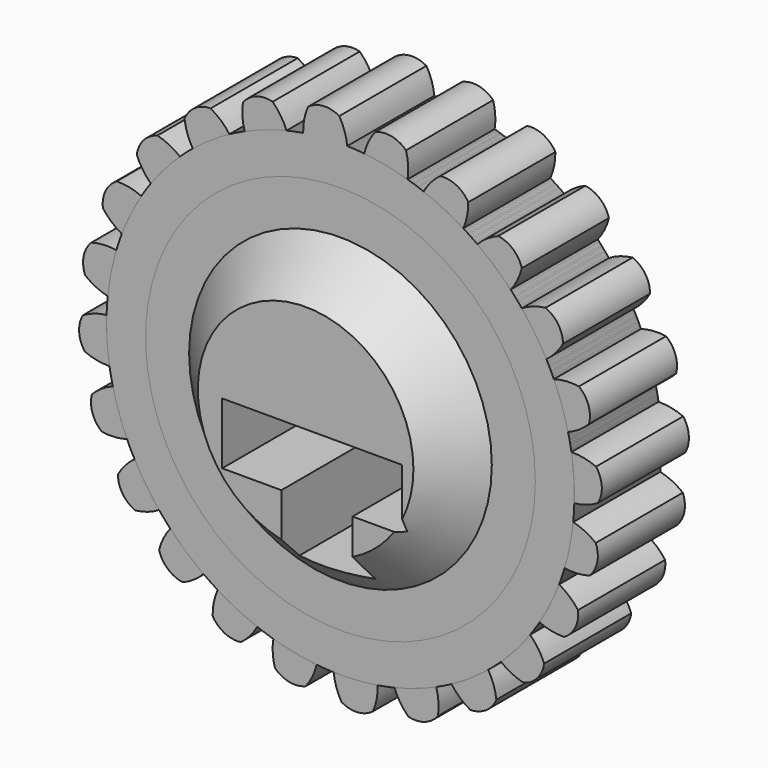
from build123d import *

# Parameters (mm, degrees)
F0_R     = 34.7544830967
F1_DEPTH = 25
F2_COUNT = 24
F3_DEPTH = 25
F4_DEPTH = 35


# Not quite as in the source:
# - a fillet or chamfer that OpenCascade refuses, or shapes differently, is made with other operations: its cross-section is extruded or revolved along the edge and cut away or added


with BuildPart() as f1:
    # F0 (on Front) → F1 (new body)
    with BuildSketch(Plane.XZ):
        with BuildLine():
            ThreePointArc((-8.5592843012, 53.0347479795), (-3.5135215054, 53.6059792153), (1.5636347284, 53.6982391465))
            ThreePointArc((1.5636347284, 53.6982391465), (0.9452694669, 56.5284341195), (-0.2671070692, 59.1595027839))
            ThreePointArc((-0.2671070692, 59.1595027839), (-3.9330463258, 60.0066910843), (-7.4570427008, 58.6882495052))
            ThreePointArc((-7.4570427008, 58.6882495052), (-8.3156238134, 55.9214431052), (-8.5592843012, 53.0347479795))
        make_face()
        with BuildLine():
            ThreePointArc((-8.5592843012, 53.0347479795), (-34.8291008286, -40.9008505593), (53.721, 0))
            ThreePointArc((53.721, 0), (38.5353465162, 37.4295726649), (1.5636347284, 53.6982391465))
            ThreePointArc((1.5636347284, 53.6982391465), (-3.5135215054, 53.6059792153), (-8.5592843012, 53.0347479795))
        make_face()
        Circle(F0_R, mode=Mode.SUBTRACT)
    extrude(amount=F1_DEPTH)


with BuildPart() as f2_1:
    # F2: instance of F1
    add(f1.part.rotate(Axis((0, 0, 0), (0, 1, 0)), 1 * 360 / F2_COUNT))


with BuildPart() as f2_2:
    # F2: instance of F1
    add(f1.part.rotate(Axis((0, 0, 0), (0, 1, 0)), 2 * 360 / F2_COUNT))


with BuildPart() as f2_3:
    # F2: instance of F1
    add(f1.part.rotate(Axis((0, 0, 0), (0, 1, 0)), 3 * 360 / F2_COUNT))


with BuildPart() as f2_4:
    # F2: instance of F1
    add(f1.part.rotate(Axis((0, 0, 0), (0, 1, 0)), 4 * 360 / F2_COUNT))


with BuildPart() as f2_5:
    # F2: instance of F1
    add(f1.part.rotate(Axis((0, 0, 0), (0, 1, 0)), 5 * 360 / F2_COUNT))


with BuildPart() as f2_6:
    # F2: instance of F1
    add(f1.part.rotate(Axis((0, 0, 0), (0, 1, 0)), 6 * 360 / F2_COUNT))


with BuildPart() as f2_7:
    # F2: instance of F1
    add(f1.part.rotate(Axis((0, 0, 0), (0, 1, 0)), 7 * 360 / F2_COUNT))


with BuildPart() as f2_8:
    # F2: instance of F1
    add(f1.part.rotate(Axis((0, 0, 0), (0, 1, 0)), 8 * 360 / F2_COUNT))


with BuildPart() as f2_9:
    # F2: instance of F1
    add(f1.part.rotate(Axis((0, 0, 0), (0, 1, 0)), 9 * 360 / F2_COUNT))


with BuildPart() as f2_10:
    # F2: instance of F1
    add(f1.part.rotate(Axis((0, 0, 0), (0, 1, 0)), 10 * 360 / F2_COUNT))


with BuildPart() as f2_11:
    # F2: instance of F1
    add(f1.part.rotate(Axis((0, 0, 0), (0, 1, 0)), 11 * 360 / F2_COUNT))


with BuildPart() as f2_12:
    # F2: instance of F1
    add(f1.part.rotate(Axis((0, 0, 0), (0, 1, 0)), 12 * 360 / F2_COUNT))


with BuildPart() as f2_13:
    # F2: instance of F1
    add(f1.part.rotate(Axis((0, 0, 0), (0, 1, 0)), 13 * 360 / F2_COUNT))


with BuildPart() as f2_14:
    # F2: instance of F1
    add(f1.part.rotate(Axis((0, 0, 0), (0, 1, 0)), 14 * 360 / F2_COUNT))


with BuildPart() as f2_15:
    # F2: instance of F1
    add(f1.part.rotate(Axis((0, 0, 0), (0, 1, 0)), 15 * 360 / F2_COUNT))


with BuildPart() as f2_16:
    # F2: instance of F1
    add(f1.part.rotate(Axis((0, 0, 0), (0, 1, 0)), 16 * 360 / F2_COUNT))


with BuildPart() as f2_17:
    # F2: instance of F1
    add(f1.part.rotate(Axis((0, 0, 0), (0, 1, 0)), 17 * 360 / F2_COUNT))


with BuildPart() as f2_18:
    # F2: instance of F1
    add(f1.part.rotate(Axis((0, 0, 0), (0, 1, 0)), 18 * 360 / F2_COUNT))


with BuildPart() as f2_19:
    # F2: instance of F1
    add(f1.part.rotate(Axis((0, 0, 0), (0, 1, 0)), 19 * 360 / F2_COUNT))


with BuildPart() as f2_20:
    # F2: instance of F1
    add(f1.part.rotate(Axis((0, 0, 0), (0, 1, 0)), 20 * 360 / F2_COUNT))


with BuildPart() as f2_21:
    # F2: instance of F1
    add(f1.part.rotate(Axis((0, 0, 0), (0, 1, 0)), 21 * 360 / F2_COUNT))


with BuildPart() as f2_22:
    # F2: instance of F1
    add(f1.part.rotate(Axis((0, 0, 0), (0, 1, 0)), 22 * 360 / F2_COUNT))


with BuildPart() as f2_23:
    # F2: instance of F1
    add(f1.part.rotate(Axis((0, 0, 0), (0, 1, 0)), 23 * 360 / F2_COUNT))


with BuildPart() as f3:
    # F0 (on Front) → F3 (new body)
    with BuildSketch(Plane.XZ):
        with BuildLine():
            ThreePointArc((-8.5592843012, 53.0347479795), (-34.8291008286, -40.9008505593), (53.721, 0))
            ThreePointArc((53.721, 0), (38.5353465162, 37.4295726649), (1.5636347284, 53.6982391465))
            ThreePointArc((1.5636347284, 53.6982391465), (-3.5135215054, 53.6059792153), (-8.5592843012, 53.0347479795))
        make_face()
        Circle(F0_R, mode=Mode.SUBTRACT)
        with BuildLine():
            ThreePointArc((-8.5592843012, 53.0347479795), (-3.5135215054, 53.6059792153), (1.5636347284, 53.6982391465))
            ThreePointArc((1.5636347284, 53.6982391465), (0.9452694669, 56.5284341195), (-0.2671070692, 59.1595027839))
            ThreePointArc((-0.2671070692, 59.1595027839), (-3.9330463258, 60.0066910843), (-7.4570427008, 58.6882495052))
            ThreePointArc((-7.4570427008, 58.6882495052), (-8.3156238134, 55.9214431052), (-8.5592843012, 53.0347479795))
        make_face()
        Circle(F0_R)
        Polygon((-19.1621500999, -14.1272554174), (-19.1621500999, 0), (22.1784766763, 0), (22.1784766763, -14.12726), (10.7779512182, -14.12726), (10.7779512182, -29.45111), (-5.5678868666, -29.4511094689), (-5.5678868666, -14.1272554174), align=None, mode=Mode.SUBTRACT)
    extrude(amount=F3_DEPTH)


with BuildPart() as f4:
    # F0 (on Front) → F4 (new body)
    with BuildSketch(Plane.XZ):
        Circle(F0_R)
        Polygon((-19.1621500999, -14.1272554174), (-19.1621500999, 0), (22.1784766763, 0), (22.1784766763, -14.12726), (10.7779512182, -14.12726), (10.7779512182, -29.45111), (-5.5678868666, -29.4511094689), (-5.5678868666, -14.1272554174), align=None, mode=Mode.SUBTRACT)
    extrude(amount=F4_DEPTH)

    # F5#2: chamfer of 10 on 1 edges, made by hand

    # F5_2_s1 → F5_2_t2 (revolve, cut)
    with BuildSketch(Plane.XY):
        Polygon((34.7544830967, -25), (24.7544830967, -35), (34.7544830967, -35), align=None)
    revolve(axis=Axis((0, -35, 0), (0, -1, 0)), mode=Mode.SUBTRACT)


with BuildPart() as f1_1:
    add(f1.part)

    # F5: chamfer of 10 on 1 edges, made by hand

    # F5_s1 → F5_t2 (revolve, cut)
    with BuildSketch(Plane.XY):
        Polygon((34.7544830967, -15), (44.7544830967, -25), (34.7544830967, -25), align=None)
    revolve(axis=Axis((0, -25, 0), (0, -1, 0)), mode=Mode.SUBTRACT)


solid = Compound([f2_1.part, f2_2.part, f2_3.part, f2_4.part, f2_5.part, f2_6.part, f2_7.part, f2_8.part, f2_9.part, f2_10.part, f2_11.part, f2_12.part, f2_13.part, f2_14.part, f2_15.part, f2_16.part, f2_17.part, f2_18.part, f2_19.part, f2_20.part, f2_21.part, f2_22.part, f2_23.part, f3.part, f4.part, f1_1.part])
